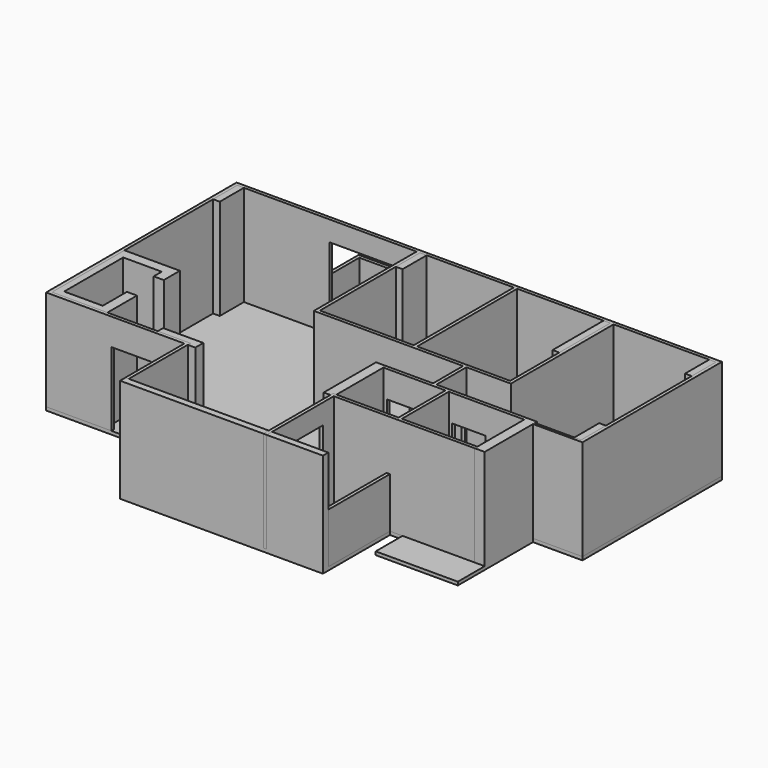
from build123d import *

# Parameters (mm, degrees)
F1_DEPTH  = 100
F3_DEPTH  = 3000
F4_W      = 300
F4_H      = 1000
F4_H_2    = 2000
F4_H_3    = 1950
F4_W_2    = 1200
F4_H_4    = 300
F4_W_3    = 6050
F4_H_5    = 200
F5_DEPTH  = 3000
F6_W      = 2750
F6_H      = 100
F7_DEPTH  = 3000
F8_W      = 2800
F8_H      = 3730
F8_W_2    = 2775
F9_DEPTH  = 3000
F10_W     = 1200
F10_H     = 2200
F11_DEPTH = 100
F12_W     = 1000
F12_H     = 2200
F13_DEPTH = 100
F14_W     = 1000
F14_H     = 2200
F15_DEPTH = 100
F16_W     = 1000
F16_H     = 2200
F17_DEPTH = 100
F18_W     = 1600
F18_H     = 2400
F19_DEPTH = 100
F20_W     = 2300
F20_H     = 2400
F21_DEPTH = 100
F22_W     = 100
F22_H     = 2300
F23_DEPTH = 1500


with BuildPart() as f1:
    # F0 (on Top) → F1 (new body)
    with BuildSketch(Plane.XY):
        Polygon((-4125, 0), (0, 0), (0, -2400), (6050, -2400), (6050, -900), (6050, 0), (6050, 100), (6425, 100), (6425, 0), (6425, -900), (8875, -900), (8875, 1900), (10350, 1900), (10350, 7100), (1175, 7100), (1175, 8275), (-1425, 8275), (-1425, 7100), (-4125, 7100), align=None)
    extrude(amount=-F1_DEPTH)

    # F2 (on face) → F3 (join)
    with BuildSketch(Plane.XY):
        Polygon((-4125, 2800), (-4125, 0), (-2375, 0), (-2375, 1200), (-2675, 1200), (-2675, 300), (-3825, 300), (-3825, 2500), (-2675, 2500), (-2675, 2200), (-2375, 2200), (-2375, 2800), align=None)
    extrude(amount=F3_DEPTH)

    # F4 (on face) → F5 (join)
    with BuildSketch(Plane.XY):
        with Locations((-3975, 6600)):
            Rectangle(F4_W, F4_H)
        with Locations((1475, 6600)):
            Rectangle(F4_W, F4_H)
        with Locations((7050, 6100)):
            Rectangle(F4_W, F4_H_2)
        with Locations((10200, 6600)):
            Rectangle(F4_W, F4_H)
        with Locations((10200, 2400)):
            Rectangle(F4_W, F4_H)
        with Locations((8725, 1075)):
            Rectangle(F4_W, F4_H_3)
        with Locations((4225, 1075)):
            Rectangle(F4_W, F4_H_3)
        with Locations((-275, 150)):
            Rectangle(F4_W_2, F4_H_4)
        with Locations((3025, -2300)):
            Rectangle(F4_W_3, F4_H_5)
    extrude(amount=F5_DEPTH)


with BuildPart() as f7:
    # F6 (on face) → F7 (new body)
    with BuildSketch(Plane.XY):
        Polygon((0, 0), (0, -2200), (100, -2200), (100, 100), (-4025, 100), (-4025, 7000), (-1425, 7000), (-1425, 7100), (-4125, 7100), (-4125, 0), align=None)
        with Locations((-50, 7050)):
            Rectangle(F6_W, F6_H)
    extrude(amount=F7_DEPTH)

    # F8 (on face) → F9 (join)
    with BuildSketch(Plane.XY):
        Polygon((5875, 3170), (7200, 3170), (7200, 7000), (7200, 7100), (1325, 7100), (1325, 3170), (5775, 3170), (5775, 2050), (4375, 2050), (4375, 1950), (6225, 1950), (6225, 200), (4375, 200), (4375, 100), (8575, 100), (8575, 200), (6325, 200), (6325, 1950), (8575, 1950), (8575, 2050), (5875, 2050), align=None)
        with Locations((2825, 5135)):
            Rectangle(F8_W, F8_H, mode=Mode.SUBTRACT)
        with Locations((5712.5, 5135)):
            Rectangle(F8_W_2, F8_H, mode=Mode.SUBTRACT)
        Polygon((7200, 7100), (7200, 7000), (10250, 7000), (10250, 1975), (8875, 1975), (8875, 1900), (10250, 1900), (10350, 1900), (10350, 7000), (10350, 7100), (10250, 7100), align=None)
        Polygon((4375, -2400), (4375, 100), (4375, 200), (4275, 200), (4275, -2400), align=None)
    extrude(amount=F9_DEPTH)

    # F10 (on face) → F11 (cut)
    with BuildSketch(Plane.XZ):
        with Locations((-1575, 1100)):
            Rectangle(F10_W, F10_H)
    extrude(amount=-F11_DEPTH, mode=Mode.SUBTRACT)

    # F12 (on face) → F13 (cut)
    with BuildSketch(Plane.XZ.offset(-3170)):
        with Locations((3675, 1100)):
            Rectangle(F12_W, F12_H)
        with Locations((4975, 1100)):
            Rectangle(F12_W, F12_H)
    extrude(amount=-F13_DEPTH, mode=Mode.SUBTRACT)

    # F14 (on face) → F15 (cut)
    with BuildSketch(Plane(origin=(5775, 0, 0), x_dir=(0, -1, 0), z_dir=(-1, 0, 0))):
        with Locations((-2610, 1100)):
            Rectangle(F14_W, F14_H)
    extrude(amount=-F15_DEPTH, mode=Mode.SUBTRACT)

    # F16 (on face) → F17 (cut)
    with BuildSketch(Plane(origin=(0, 2050, 0), x_dir=(-1, 0, 0), z_dir=(0, 1, 0))):
        with Locations((-4975, 1100)):
            Rectangle(F16_W, F16_H)
        with Locations((-6925, 1100)):
            Rectangle(F16_W, F16_H)
    extrude(amount=-F17_DEPTH, mode=Mode.SUBTRACT)

    # F18 (on face) → F19 (cut)
    with BuildSketch(Plane(origin=(4275, 0, 0), x_dir=(0, -1, 0), z_dir=(-1, 0, 0))):
        with Locations((1100, 1200)):
            Rectangle(F18_W, F18_H)
    extrude(amount=-F19_DEPTH, mode=Mode.SUBTRACT)

    # F20 (on face) → F21 (cut)
    with BuildSketch(Plane.XZ.offset(-7000)):
        with Locations((-125, 1200)):
            Rectangle(F20_W, F20_H)
    extrude(amount=-F21_DEPTH, mode=Mode.SUBTRACT)

    # F22 (on face) → F23 (join)
    with BuildSketch(Plane.XY):
        Polygon((-1425, 8275), (-1425, 7100), (-1325, 7100), (-1325, 8175), (1075, 8175), (1075, 7100), (1175, 7100), (1175, 8275), align=None)
        with Locations((6000, -1050)):
            Rectangle(F22_W, F22_H)
    extrude(amount=F23_DEPTH)


solid = Compound([f1.part, f7.part])
